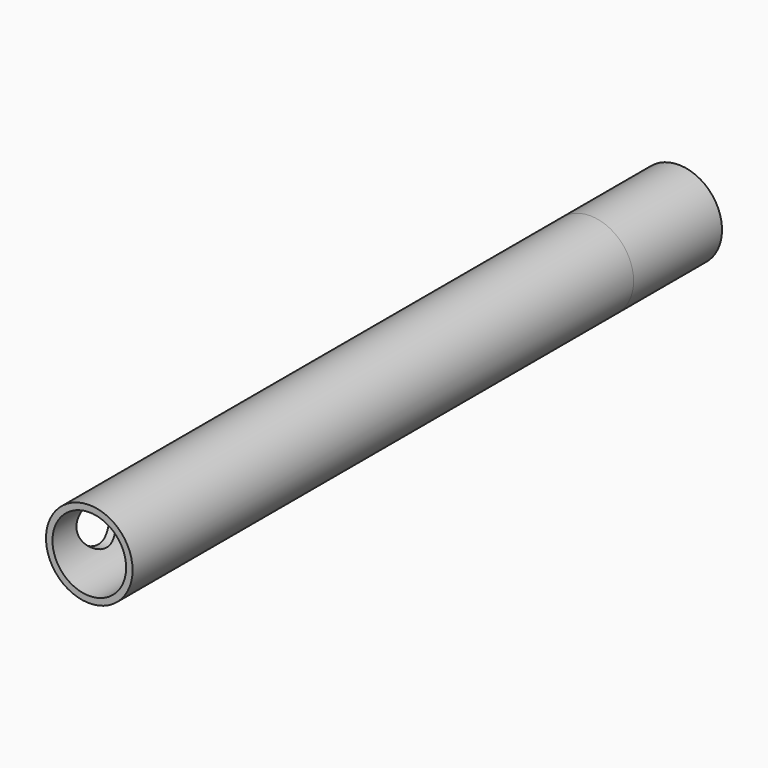
from build123d import *

# Parameters (mm, degrees)
F3_R      = 4.7
F4_DEPTH  = 43
F8_DEPTH  = 43
F6_R      = 4.7
F6_R_2    = 4
F9_DEPTH  = 25
F7_R      = 4.7
F7_R_2    = 4
F10_DEPTH = 12
F11_R     = 2.75
F12_DEPTH = 4.701


# Not quite as in the source:
# - ends of sketch curves that miss each other by under 0.0002 mm in the source are joined


with BuildPart() as f4:
    # F3 (on Front) → F4 (new body)
    with BuildSketch(Plane.XZ):
        Circle(F3_R)
    extrude(amount=F4_DEPTH)

    # F5 (on face) → F8 (cut, through all)
    with BuildSketch(Plane.XZ.offset(43)):
        with BuildLine():
            Line((-1.25, -3.8), (0, -3.8))
            Line((0, -3.8), (1.25, -3.8))
            Line((1.25, -3.8), (1.25, -3.7))
            ThreePointArc((1.25, -3.7), (1.3085786438, -3.5585786438), (1.45, -3.5))
            Line((1.45, -3.5), (2, -3.5))
            Line((2, -3.5), (2, -3.05))
            ThreePointArc((2, -3.05), (2.0585786438, -2.9085786438), (2.2, -2.85))
            Line((2.2, -2.85), (3.15, -2.85))
            Line((3.15, -2.85), (3.15, -2.15))
            Line((3.15, -2.15), (2.2, -2.15))
            ThreePointArc((2.2, -2.15), (2.0585786438, -2.0914213562), (2, -1.95))
            Line((2, -1.95), (2, -1.887459))
            ThreePointArc((2, -1.887459), (2.1033535752, -1.771554046), (2.2, -1.65))
            Line((2.2, -1.65), (3.75, -1.65))
            Line((3.75, -1.65), (3.75, 0))
            Line((3.75, 0), (3.75, 1.65))
            Line((3.75, 1.65), (2.2, 1.65))
            ThreePointArc((2.2, 1.65), (2.1033535752, 1.771554046), (1.9999998047, 1.8874588157))
            Line((1.9999998047, 1.8874588157), (2, 1.95))
            ThreePointArc((2, 1.95), (2.0585786438, 2.0914213562), (2.2, 2.15))
            Line((2.2, 2.15), (3.15, 2.15))
            Line((3.15, 2.15), (3.15, 2.85))
            Line((3.15, 2.85), (2.2, 2.85))
            ThreePointArc((2.2, 2.85), (2.0585786438, 2.9085786438), (2, 3.05))
            Line((2, 3.05), (2, 3.5))
            Line((2, 3.5), (1.45, 3.5))
            ThreePointArc((1.45, 3.5), (1.3085786438, 3.5585786438), (1.25, 3.7))
            Line((1.25, 3.7), (1.25, 3.8))
            Line((1.25, 3.8), (0, 3.8))
            Line((0, 3.8), (-1.25, 3.8))
            Line((-1.25, 3.8), (-1.25, 3.7))
            ThreePointArc((-1.25, 3.7), (-1.3085786438, 3.5585786438), (-1.45, 3.5))
            Line((-1.45, 3.5), (-2, 3.5))
            Line((-2, 3.5), (-2, 3.05))
            ThreePointArc((-2, 3.05), (-2.0585786438, 2.9085786438), (-2.2, 2.85))
            Line((-2.2, 2.85), (-3.15, 2.85))
            Line((-3.15, 2.85), (-3.15, 2.15))
            Line((-3.15, 2.15), (-2.2, 2.15))
            ThreePointArc((-2.2, 2.15), (-2.0585786438, 2.0914213562), (-2, 1.95))
            Line((-2, 1.95), (-2, 1.887459))
            ThreePointArc((-2, 1.887459), (-2.1033535752, 1.771554046), (-2.2, 1.65))
            Line((-2.2, 1.65), (-3.75, 1.65))
            Line((-3.75, 1.65), (-3.75, 0))
            Line((-3.75, 0), (-3.75, -1.65))
            Line((-3.75, -1.65), (-2.2, -1.65))
            ThreePointArc((-2.2, -1.65), (-2.1033535752, -1.771554046), (-1.9999998047, -1.8874588157))
            Line((-1.9999998047, -1.8874588157), (-2, -1.95))
            ThreePointArc((-2, -1.95), (-2.0585786438, -2.0914213562), (-2.2, -2.15))
            Line((-2.2, -2.15), (-3.15, -2.15))
            Line((-3.15, -2.15), (-3.15, -2.85))
            Line((-3.15, -2.85), (-2.2, -2.85))
            ThreePointArc((-2.2, -2.85), (-2.0585786438, -2.9085786438), (-2, -3.05))
            Line((-2, -3.05), (-2, -3.5))
            Line((-2, -3.5), (-1.45, -3.5))
            ThreePointArc((-1.45, -3.5), (-1.3085786438, -3.5585786438), (-1.25, -3.7))
            Line((-1.25, -3.7), (-1.25, -3.8))
        make_face()
    extrude(amount=-F8_DEPTH, mode=Mode.SUBTRACT)

    # F6 (on face) → F9 (join)
    with BuildSketch(Plane.XZ.offset(43)):
        Circle(F6_R)
        Circle(F6_R_2, mode=Mode.SUBTRACT)
    extrude(amount=F9_DEPTH)

    # F7 (on face) → F10 (join)
    with BuildSketch(Plane(origin=(0, 0, 0), x_dir=(-1, 0, 0), z_dir=(0, 1, 0))):
        Circle(F7_R)
        Circle(F7_R_2, mode=Mode.SUBTRACT)
    extrude(amount=F10_DEPTH)

    # F11 (on Right) → F12 (cut, through all)
    with BuildSketch(Plane.YZ):
        with Locations((-62, 0)):
            Circle(F11_R)
    extrude(amount=-F12_DEPTH, mode=Mode.SUBTRACT)


solid = f4.part
